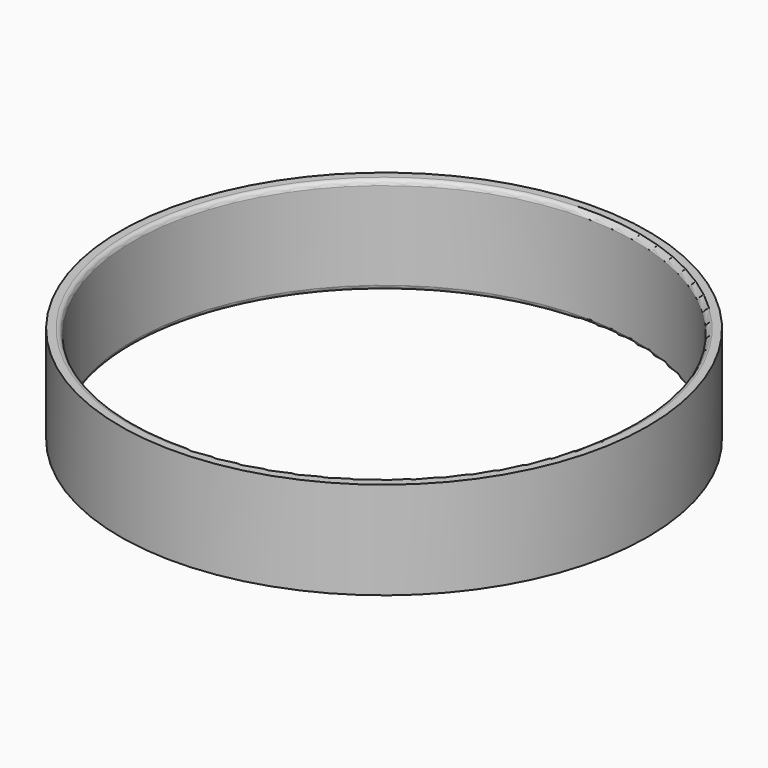
from build123d import *

# Parameters (mm, degrees)
F0_R     = 27.1
F0_R_2   = 25.8
F1_DEPTH = 10
F2_R     = 0.5


# Not quite as in the source:
# - a feature names something its author has since deleted; it is built from what else it names


with BuildPart() as f1:
    # F0 (on Top) → F1 (new body)
    with BuildSketch(Plane.XY):
        Circle(F0_R)
        Circle(F0_R_2, mode=Mode.SUBTRACT)
    extrude(amount=-F1_DEPTH)

    # F2
    f2_edges = [f1.edges().sort_by_distance(p)[0] for p in [
        (-25.8, 0, 0),
        (-25.8, 0, -10),
    ]]
    fillet(f2_edges, radius=F2_R)


solid = f1.part
